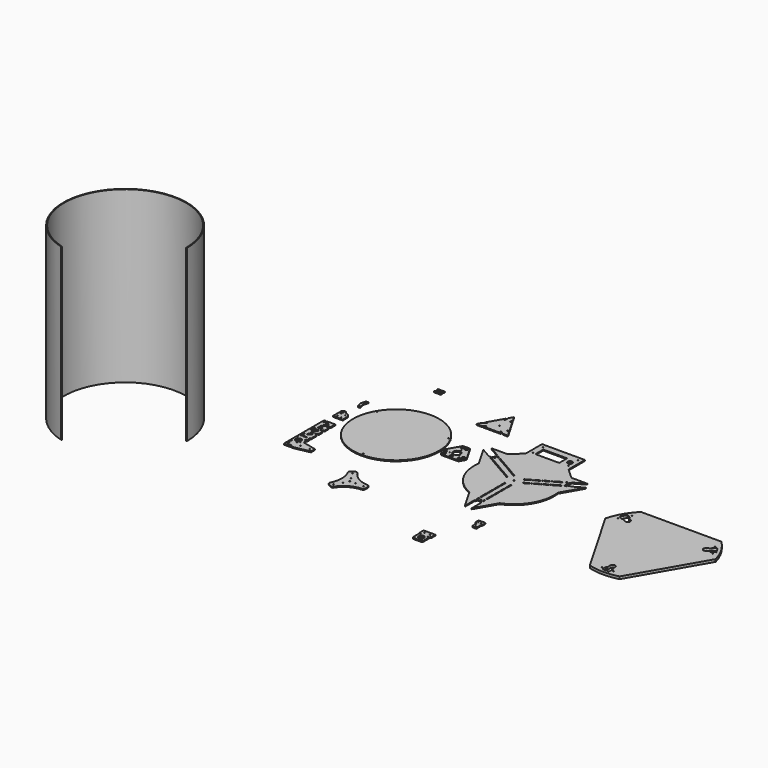
from build123d import *

# Parameters (mm, degrees)
F0_R      = 1.49999625
F0_R_2    = 1.999995
F0_R_3    = 11.4999712501
F0_W      = 3.999994
F0_H      = 4.6031024922
F0_R_4    = 4.49998875
F1_DEPTH  = 4
F0_R_5    = 177.4995562511
F0_W_2    = 3.99999
F0_H_2    = 9.9561866095
F0_R_6    = 2
F0_W_3    = 19.9999510001
F0_H_3    = 3.4640928398
F0_W_4    = 3.999988
F0_H_4    = 7.9999760001
F0_R_7    = 1.9999942213
F0_W_5    = 4
F0_H_5    = 29.9999350002
F0_H_6    = 19.9999400001
F0_H_7    = 19.9999410001
F0_H_8    = 23.1915490211
F0_R_8    = 2.4999934422
F0_R_9    = 1.9999957017
F0_R_10   = 1.75
F0_R_11   = 1.9999950064
F0_R_12   = 10
F0_R_13   = 1.9999769978
F0_R_14   = 1.9999882693
F0_R_15   = 2.0033655233
F0_R_16   = 1.4940821477
F0_R_17   = 1.9930891667
F2_R      = 2
F2_R_2    = 1.5
F3_DEPTH  = 4
F4_R      = 5.9
F4_R_2    = 1.5
F4_R_3    = 6
F4_R_4    = 15
F5_DEPTH  = 4
F7_DEPTH  = 40
F9_DEPTH  = 700
F10_R     = 2
F11_DEPTH = 10
F12_R     = 1.5
F12_R_2   = 2
F14_DEPTH = 4
F13_R     = 1.6499986081
F13_R_2   = 11.0499960842
F13_R_3   = 2


# Not quite as in the source:
# - ends of sketch curves that miss each other by under 0.0002 mm in the source are joined


with BuildPart() as f1:
    # F0 (on Top) → F1 (new body)
    with BuildSketch(Plane.XY):
        Polygon((-439.5795490511, -125.5086882283), (-439.6210259474, -125.4915762711), (-440.7988980027, -125.4915762711), (-440.7988980027, -122.491583771), (-439.1989020027, -122.491583771), (-439.1989020027, -122.5621985945), (-439.1938570154, -122.5615335962), (-439.1955270112, -120.5603685991), (-435.9955370112, -120.5576966058), (-435.9938640153, -122.5615335962), (-432.9989175027, -122.5615335962), (-432.9989175027, -118.6865432836), (-428.9989275027, -118.6865432836), (-428.9989275027, -95.4949932625), (-464.8342439144, -95.4949932625), (-464.8342439144, -106.9297106757), (-468.8342339144, -106.9297106757), (-468.8342339144, -95.4949932625), (-474.998812503, -95.4949932625), (-474.998812503, -302.9560376099), (-432.9989175027, -302.9560376099), (-372.9990675023, -290.4291429271), (-372.9990675023, -270.429192927), (-428.9989275027, -257.2412538969), (-428.9989275027, -249.2412738968), (-432.9989175027, -249.2412738968), (-432.9989175027, -238.816799958), (-428.9989275027, -238.816799958), (-428.9989275027, -230.8168199579), (-432.9989175027, -230.8168199579), (-432.9989175027, -220.9362876593), (-428.9989275027, -220.9362876593), (-428.9989275027, -190.9363626591), (-432.9989175027, -190.9363626591), (-432.9989175027, -187.0613723466), (-435.9400231499, -187.0563143592), (-435.9441941395, -189.0601753496), (-439.1441871395, -189.0601753496), (-439.1400291499, -187.0664223339), (-440.7322311694, -187.0664223339), (-440.7322311694, -184.0664298339), (-439.1808460479, -184.0664298339), (-439.1425161437, -184.0613798465), (-439.1441871395, -182.0601928495), (-435.9441941395, -182.0601928495), (-435.9425231437, -184.0613798465), (-432.9989175027, -184.0613798465), (-432.9989175027, -180.186389534), (-428.9989275027, -180.186389534), (-428.9989275027, -160.1864395339), (-432.9989175027, -160.1864395339), (-432.9989175027, -156.3114492214), (-435.9656930858, -156.306413234), (-435.9640200899, -158.3102612243), (-439.16401409, -158.3102612243), (-439.1656840858, -156.3090842273), (-439.236808908, -156.2998332504), (-440.7655640861, -156.2998332504), (-440.7655640861, -153.2998407504), (-439.1681960795, -153.2998407504), (-439.1698570754, -151.3102807243), (-435.9698640753, -151.3102807243), (-435.9681930795, -153.3114567214), (-432.9989175027, -153.3114567214), (-432.9989175027, -149.4364664088), (-428.9989275027, -149.4364664088), (-428.9989275027, -129.4365164087), (-432.9989175027, -129.4365164087), (-432.9989175027, -125.5615260962), (-435.9913630216, -125.5565111087), (-435.9896930258, -127.5576771058), (-439.1896840258, -127.5603480991), (-439.1913540216, -125.559183102), align=None)
        with BuildLine():
            add(Edge.make_bspline(
                [(-445.5863090342, -297.4957282607), (-445.5863090342, -294.0828727047), (-459.7051392371, -295.7893004827), (-473.8239694401, -297.4957282607), (-459.7051392371, -299.2021560387), (-445.5863090342, -300.9085838167), (-445.5863090342, -297.4957282607)],
                knots=[0, 0, 0, 2.0943951024, 2.0943951024, 4.1887902048, 4.1887902048, 6.2831853072, 6.2831853072, 6.2831853072], degree=2, weights=[1, 0.5, 1, 0.5, 1, 0.5, 1]))
        make_face(mode=Mode.SUBTRACT)
        with Locations((-469.552397119, -291.3865105337)):
            Circle(F0_R, mode=Mode.SUBTRACT)
        with Locations((-438.4448498879, -291.3865105337)):
            Circle(F0_R, mode=Mode.SUBTRACT)
        with Locations((-469.4988262529, -280.6365374087)):
            Circle(F0_R_2, mode=Mode.SUBTRACT)
        with Locations((-469.5517851205, -268.9985985035)):
            Circle(F0_R, mode=Mode.SUBTRACT)
        with Locations((-448.2801512996, -268.9919315202)):
            Circle(F0_R, mode=Mode.SUBTRACT)
        with Locations((-423.4178604553, -280.6365374087)):
            Circle(F0_R_2, mode=Mode.SUBTRACT)
        with Locations((-386.1206556984, -280.6365374087)):
            Circle(F0_R_2, mode=Mode.SUBTRACT)
        with Locations((-453.844811388, -253.5207241982)):
            Circle(F0_R_3, mode=Mode.SUBTRACT)
        with Locations((-439.7278266804, -262.5266596833)):
            Circle(F0_R, mode=Mode.SUBTRACT)
        with Locations((-469.5258531854, -237.9090702273)):
            Circle(F0_R, mode=Mode.SUBTRACT)
        with Locations((-438.4448498879, -237.9631240922)):
            Circle(F0_R, mode=Mode.SUBTRACT)
        with Locations((-467.4761833095, -222.8868237829)):
            Rectangle(F0_W, F0_H, mode=Mode.SUBTRACT)
        with BuildLine():
            add(Edge.make_bspline(
                [(-442.6737393156, -222.7585111037), (-442.6737393156, -219.3456555477), (-456.7925695186, -221.0520833257), (-470.9113997215, -222.7585111037), (-456.7925695186, -224.4649388817), (-442.6737393156, -226.1713666597), (-442.6737393156, -222.7585111037)],
                knots=[0, 0, 0, 2.0943951024, 2.0943951024, 4.1887902048, 4.1887902048, 6.2831853072, 6.2831853072, 6.2831853072], degree=2, weights=[1, 0.5, 1, 0.5, 1, 0.5, 1]))
        make_face(mode=Mode.SUBTRACT)
        with Locations((-467.4988312529, -214.9663525841)):
            Circle(F0_R, mode=Mode.SUBTRACT)
        Polygon((-469.4761793095, -205.1884330289), (-465.4761863095, -205.1884330289), (-465.4761863095, -209.8352954118), (-469.4761803095, -209.8352954118), align=None, mode=Mode.SUBTRACT)
        Polygon((-451.9988700028, -205.9363251592), (-461.4988462529, -205.9363251592), (-452.1737155657, -195.9363501591), (-451.9988700028, -195.9363501591), (-451.9814170465, -195.7301356747), (-447.2921947695, -190.7015612461), (-442.4988937528, -195.9363501591), align=None, mode=Mode.SUBTRACT)
        with Locations((-451.9988700028, -185.5664260839)):
            Circle(F0_R_4, mode=Mode.SUBTRACT)
        Polygon((-465.5654720863, -167.7282536794), (-465.5654720863, -172.3313561716), (-469.5654650863, -172.3313561716), (-469.5654660863, -167.7282536794), align=None, mode=Mode.SUBTRACT)
        with Locations((-467.5654690863, -162.2343414141)):
            Circle(F0_R, mode=Mode.SUBTRACT)
        Polygon((-456.7275011812, -180.397214007), (-461.4988462529, -175.186402034), (-451.9988700028, -165.1864270339), (-461.4988462529, -165.1864270339), (-456.7488581278, -159.9989750026), (-447.3363046592, -159.9989750026), (-442.6737393156, -165.1864270339), align=None, mode=Mode.SUBTRACT)
        Polygon((-469.5654650863, -152.3314141715), (-465.5654720863, -152.3314141715), (-465.5654720863, -156.9782765543), (-469.5654660863, -156.9782765543), align=None, mode=Mode.SUBTRACT)
        Polygon((-456.7055452361, -129.2017149957), (-442.4988937528, -144.4364789088), (-447.2488818778, -149.62400094), (-456.7488581278, -149.62400094), (-461.4988462529, -144.4364789088), (-451.9988700028, -144.4364789088), (-461.4988462529, -134.4365039087), align=None, mode=Mode.SUBTRACT)
        with Locations((-451.9988700028, -123.991580021)):
            Circle(F0_R_4, mode=Mode.SUBTRACT)
        Polygon((-451.8240234399, -103.6865807835), (-442.4988937528, -113.6865557836), (-447.2921947695, -118.9213456966), (-461.4988462529, -103.6865807835), align=None, mode=Mode.SUBTRACT)
    extrude(amount=F1_DEPTH)


with BuildPart() as f1b:
    # F0 (on Top) → F1, piece 2 (new body)
    with BuildSketch(Plane.XY):
        with Locations((-231.1251601871, -29.9759380602)):
            Circle(F0_R_5)
        with Locations((-231.1251601871, -199.2255149362)):
            Circle(F0_R_2, mode=Mode.SUBTRACT)
        with Locations((-378.5313116717, 55.8541043647)):
            Circle(F0_R_2, mode=Mode.SUBTRACT)
        with Locations((-83.6997907505, 56.0153949615)):
            Circle(F0_R_2, mode=Mode.SUBTRACT)
    extrude(amount=F1_DEPTH)


with BuildPart() as f1c:
    # F0 (on Top) → F1, piece 3 (new body)
    with BuildSketch(Plane.XY):
        Polygon((-442.7478361304, 91.5328801678), (-451.8370994072, 91.5328801678), (-457.283592791, 71.5697730756), (-451.8370994072, 49.5329861675), (-442.7478361304, 49.5329861493), (-448.1943295142, 71.5697720756), align=None)
        with Locations((-448.8326909183, 54.9859315352)):
            Circle(F0_R, mode=Mode.SUBTRACT)
        with Locations((-448.7918990202, 86.0799338002)):
            Circle(F0_R, mode=Mode.SUBTRACT)
    extrude(amount=F1_DEPTH)


with BuildPart() as f1d:
    # F0 (on Top) → F1, piece 4 (new body)
    with BuildSketch(Plane.XY):
        Polygon((-312.8262449344, 291.4364354089), (-314.8593918515, 291.4364354089), (-314.8610558474, 289.4432753918), (-318.0610468474, 289.4459463851), (-318.0593768516, 291.4471123822), (-321.0518233704, 291.4420963948), (-321.0518233704, 287.5671060822), (-324.999187502, 287.5671060822), (-324.999187502, 282.9560946098), (-296.999187502, 282.9560946098), (-296.999187502, 287.5671060822), (-300.9465516336, 287.5671060822), (-300.9465516336, 291.4420963948), (-303.9389981525, 291.4471123822), (-303.9373281567, 289.4459463851), (-303.9431711421, 289.4459415081), (-303.9431711421, 289.4432753918), (-307.1373191567, 289.4432753918), (-307.1373191567, 296.4432597708), (-307.1373191567, 296.4459268852), (-303.9431711421, 296.4459268852), (-303.9414991462, 294.4420888948), (-303.9389981525, 294.4420888948), (-300.9465516336, 294.4420888948), (-300.9465516336, 298.3170792073), (-296.999187502, 298.3170792073), (-296.999187502, 302.9560946098), (-324.999187502, 302.9560946098), (-324.999187502, 298.3171372072), (-321.0518233704, 298.3170792073), (-321.0518233704, 294.4420888948), (-318.0568758578, 294.4420888948), (-318.055203862, 296.4459268852), (-314.855212862, 296.4432548919), (-314.8568828578, 294.4420888948), (-314.8139219652, 294.4364279089), (-312.8262449344, 294.4364279089), align=None)
        Polygon((-307.1414921463, 294.4420888948), (-307.1414921463, 291.4364354089), (-309.1721300697, 291.4364354089), (-309.1721300697, 294.4364279089), (-309.1721300697, 294.4420888948), align=None, mode=Mode.SUBTRACT)
    extrude(amount=F1_DEPTH)


with BuildPart() as f1e:
    # F0 (on Top) → F1, piece 5 (new body)
    with BuildSketch(Plane.XY):
        Polygon((-1.8421003947, 285.6355719111), (-11.8420763948, 302.9560366099), (-21.8420513949, 285.6355719111), (-21.8420513949, 272.2152924618), (-1.8421003947, 272.2152924618), align=None)
        Polygon((16.4874262814, 195.434410914), (18.4874214067, 198.8985040612), (9.8651113372, 203.8765973085), (7.8651163372, 200.4125039687), align=None)
        Polygon((28.4873965199, 216.2189689089), (30.4873917815, 219.6830622923), (21.8650813373, 224.6611553471), (19.8650863373, 221.1970620073), align=None)
        with Locations((0.1578946053, 263.7731063172)):
            Rectangle(F0_W_2, F0_H_2)
        Polygon((-1.8421003947, 258.7950130125), (-1.8421003947, 268.751199622), (-21.8420513949, 268.751199622), (-21.8420513949, 258.7950130125), (-25.8420413949, 258.7950130125), (-25.8420413949, 268.751199622), (-25.8420413949, 272.2152924618), (-25.8420413949, 278.7073862315), (-62.7938540154, 214.7049692376), (-57.1715370057, 217.9510153453), (-54.1715435711, 219.6830622923), (-45.5492331269, 224.6611553471), (-43.5492381269, 221.1970630073), (-52.1715487116, 216.2189696768), (-42.1715730107, 198.8985041684), (-33.5492631268, 203.8765973085), (-31.5492681268, 200.4125049687), (-40.1715780711, 195.434411414), (-43.1715704387, 193.7023648085), (-48.7938880153, 190.4563178592), (25.1097362257, 190.4563178592), (19.4874189347, 193.7023643176), (16.4874262814, 195.434410914), (7.8651163372, 200.4125039687), (9.8651113372, 203.8765973085), (18.4874214067, 198.8985040612), (28.4873965199, 216.2189689089), (19.8650863373, 221.1970620073), (21.8650813373, 224.6611553471), (30.4873917815, 219.6830622923), (33.4873845882, 217.9510157079), (39.1097022257, 214.7049692376), (2.1578896053, 278.7073862315), (2.1578896053, 272.2152924618), (2.1578896053, 268.751199622), (2.1578896053, 258.7950130125), align=None)
        with Locations((-11.8420758948, 227.9562243465)):
            Circle(F0_R_6, mode=Mode.SUBTRACT)
        with Locations((-23.8420463949, 263.7731063172)):
            Rectangle(F0_W_2, F0_H_2)
        Polygon((-45.1715655711, 197.1664575839), (-55.1715419814, 214.4869227571), (-66.7938440154, 207.776783558), (-76.7938190155, 190.4563178592), (-56.7938680153, 190.4563178592), align=None)
        Polygon((-45.5492331269, 224.6611553471), (-54.1715435711, 219.6830622923), (-52.1715487116, 216.2189696768), (-43.5492381269, 221.1970630073), align=None)
        Polygon((-33.5492631268, 203.8765973085), (-42.1715730107, 198.8985041684), (-40.1715780711, 195.434411414), (-31.5492681268, 200.4125049687), align=None)
        Polygon((43.1096922258, 207.776782558), (31.4873892815, 214.4869222827), (21.4874140575, 197.1664574245), (33.1097162257, 190.4563178592), (53.1096672258, 190.4563178592), align=None)
        Polygon((21.4874140575, 197.1664574245), (31.4873892815, 214.4869222827), (28.4873965199, 216.2189689089), (18.4874214067, 198.8985040612), align=None)
        with Locations((-11.8420758948, 270.4832460419)):
            Rectangle(F0_W_3, F0_H_3)
        Polygon((-52.1715487116, 216.2189696768), (-55.1715419814, 214.4869227571), (-45.1715655711, 197.1664575839), (-42.1715730107, 198.8985041684), align=None)
    extrude(amount=F1_DEPTH)


with BuildPart() as f1f:
    # F0 (on Top) → F1, piece 6 (new body)
    with BuildSketch(Plane.XY):
        with BuildLine():
            Line((131.7235082388, 88.5993365017), (66.7513821215, 88.5993365017))
            Line((66.7513821215, 88.5993365017), (111.0197374507, 63.0409903975))
            Line((111.0197374507, 63.0409903975), (109.0197424506, 59.5768970578))
            Line((109.0197424506, 59.5768970578), (115.1252134995, 56.0519168039))
            Line((115.1252134995, 56.0519168039), (105.1252384995, 38.7314511051))
            Line((105.1252384995, 38.7314511051), (99.0197737631, 42.2564432926))
            Line((99.0197737631, 42.2564432926), (97.0197787631, 38.7923499528))
            Line((97.0197787631, 38.7923499528), (52.7514171215, 64.3506861233))
            Line((52.7514171215, 64.3506861233), (100.9852385369, -19.1927430181))
            ThreePointArc((100.9852385369, -19.1927430181), (121.3444904617, -123.6659645283), (201.6413278967, -193.5342051645))
            Line((201.6413278967, -193.5342051645), (249.8751493121, -277.0776343059))
            Line((249.8751493121, -277.0776343059), (249.8751493121, -225.9609400976))
            Line((249.8751493121, -225.9609400976), (253.8751393121, -225.9609400976))
            Line((253.8751393121, -225.9609400976), (253.8751393121, -218.9109567226))
            Line((253.8751393121, -218.9109567226), (273.8750893123, -218.9109567226))
            Line((273.8750893123, -218.9109567226), (273.8750893123, -225.9609400976))
            Line((273.8750893123, -225.9609400976), (277.8750793123, -225.9609400976))
            Line((277.8750793123, -225.9609400976), (277.8750793123, -277.0776343059))
            Line((277.8750793123, -277.0776343059), (326.1089007277, -193.5342051645))
            ThreePointArc((326.1089007277, -193.5342051645), (406.4100868046, -123.6684751011), (426.7649910875, -19.1927430181))
            Line((426.7649910875, -19.1927430181), (474.998812503, 64.3506861233))
            Line((474.998812503, 64.3506861233), (430.7304571739, 38.7923390192))
            Line((430.7304571739, 38.7923390192), (428.7304621738, 42.2564323589))
            Line((428.7304621738, 42.2564323589), (422.6249974375, 38.7314401714))
            Line((422.6249974375, 38.7314401714), (412.6250224374, 56.0519058702))
            Line((412.6250224374, 56.0519058702), (418.7304871738, 59.5768970578))
            Line((418.7304871738, 59.5768970578), (416.7304921738, 63.0409903975))
            Line((416.7304921738, 63.0409903975), (460.9988465029, 88.5993365017))
            Line((460.9988465029, 88.5993365017), (396.0267213856, 88.5993365017))
            Line((396.0267213856, 88.5993365017), (352.1159646784, 128.1467825174))
            Line((352.1159646784, 128.1467825174), (352.1159646784, 212.6197069883))
            Line((352.1159646784, 212.6197069883), (175.634264946, 212.6197069883))
            Line((175.634264946, 212.6197069883), (175.634264946, 128.1467825174))
            Line((175.634264946, 128.1467825174), (131.7235082388, 88.5993365017))
        make_face()
        with Locations((251.8751113122, -211.5364981588)):
            Rectangle(F0_W_4, F0_H_4, mode=Mode.SUBTRACT)
        with Locations((263.8751143122, -211.5364761588)):
            Circle(F0_R_7, mode=Mode.SUBTRACT)
        with Locations((275.8750793123, -211.5364771588)):
            Rectangle(F0_W_4, F0_H_4, mode=Mode.SUBTRACT)
        with Locations((251.8751443121, -182.65599636)):
            Rectangle(F0_W_5, F0_H_5, mode=Mode.SUBTRACT)
        with Locations((275.8750793123, -182.65599636)):
            Rectangle(F0_W_4, F0_H_5, mode=Mode.SUBTRACT)
        with Locations((251.8751443121, -162.2810432974)):
            Circle(F0_R_6, mode=Mode.SUBTRACT)
        with Locations((275.8750793123, -162.2810432974)):
            Circle(F0_R_6, mode=Mode.SUBTRACT)
        with Locations((206.4286084064, -22.0654858745)):
            Circle(F0_R_6, mode=Mode.SUBTRACT)
        Polygon((210.0834857913, -26.4850257874), (212.0834807913, -23.0209324477), (232.1679543738, -34.6167053514), (230.1679575801, -38.080800798), align=None, mode=Mode.SUBTRACT)
        Polygon((183.4532703668, -11.1100642248), (185.4532653668, -7.6459708851), (202.7737310657, -17.6459458851), (200.7737360657, -21.1100392249), align=None, mode=Mode.SUBTRACT)
        with Locations((179.798393129, -6.6905240572)):
            Circle(F0_R_6, mode=Mode.SUBTRACT)
        Polygon((222.0834571602, -5.7004653779), (224.0834521603, -2.2363720381), (244.1679225802, -13.8321504196), (242.1679275802, -17.2962427594), align=None, mode=Mode.SUBTRACT)
        with Locations((218.4285798248, -1.2809253793)):
            Circle(F0_R_6, mode=Mode.SUBTRACT)
        with Locations((251.8751443121, -146.9060877348)):
            Rectangle(F0_W_5, F0_H_6, mode=Mode.SUBTRACT)
        with Locations((275.8750793123, -146.9060877348)):
            Rectangle(F0_W_4, F0_H_6, mode=Mode.SUBTRACT)
        with Locations((251.8751443121, -131.5311201722)):
            Circle(F0_R_6, mode=Mode.SUBTRACT)
        with Locations((251.8751443121, -116.1561521096)):
            Rectangle(F0_W_5, F0_H_7, mode=Mode.SUBTRACT)
        with Locations((275.8750793123, -131.5311201722)):
            Circle(F0_R_6, mode=Mode.SUBTRACT)
        with Locations((275.8750793123, -116.1561521096)):
            Rectangle(F0_W_4, F0_H_7, mode=Mode.SUBTRACT)
        with Locations((251.8751443121, -100.781196047)):
            Circle(F0_R_6, mode=Mode.SUBTRACT)
        with Locations((275.8750793123, -100.781196047)):
            Circle(F0_R_6, mode=Mode.SUBTRACT)
        with Locations((251.8751443121, -83.8104359739)):
            Rectangle(F0_W_5, F0_H_8, mode=Mode.SUBTRACT)
        with Locations((275.8750793123, -83.8104359739)):
            Rectangle(F0_W_4, F0_H_8, mode=Mode.SUBTRACT)
        with Locations((263.8751148122, -41.3758700603)):
            Circle(F0_R_8, mode=Mode.SUBTRACT)
        Polygon((283.5823070442, -13.8321504196), (303.666778833, -2.2363754091), (305.6667738331, -5.7004677488), (285.5823020442, -17.2962427594), align=None, mode=Mode.SUBTRACT)
        Polygon((295.5822770443, -34.6167084582), (315.6667488331, -23.0209324477), (317.6667438331, -26.4850257874), (297.5822720443, -38.080800798), align=None, mode=Mode.SUBTRACT)
        with Locations((321.3216211994, -22.0654858423)):
            Circle(F0_R_6, mode=Mode.SUBTRACT)
        with Locations((309.3216511993, -1.2809283037)):
            Circle(F0_R_6, mode=Mode.SUBTRACT)
        Polygon((326.9764935588, -21.1100392249), (324.9764985587, -17.6459458851), (342.2969632576, -7.6459708851), (344.2969582576, -11.1100642248), align=None, mode=Mode.SUBTRACT)
        with Locations((347.9518356204, -6.6905242737)):
            Circle(F0_R_6, mode=Mode.SUBTRACT)
        Polygon((114.9758125605, 33.0442053895), (112.9758175605, 29.5801120497), (106.0476318809, 33.5801020497), (108.0476268809, 37.0441953895), align=None, mode=Mode.SUBTRACT)
        with Locations((116.5117067207, 43.7044327389)):
            Circle(F0_R_9, mode=Mode.SUBTRACT)
        Polygon((123.5326041685, 28.1039387402), (149.5133012167, 13.1039772401), (147.5133062167, 9.6398839003), (121.5326091685, 24.6398464004), align=None, mode=Mode.SUBTRACT)
        with Locations((153.1681786016, 8.6844373271)):
            Circle(F0_R_6, mode=Mode.SUBTRACT)
        Polygon((176.1435156412, -2.2709843225), (174.1435206412, -5.7350776623), (156.8230559424, 4.2648973378), (158.8230509424, 7.7289906775), align=None, mode=Mode.SUBTRACT)
        with Locations((165.1681505852, 29.4689988013)):
            Circle(F0_R_6, mode=Mode.SUBTRACT)
        Polygon((197.4532363669, 13.1385871535), (214.7737010657, 3.1386121535), (212.7737075016, -0.3254786258), (195.4532413669, 9.6744938138), align=None, mode=Mode.SUBTRACT)
        with Locations((191.79836558, 14.0940364945)):
            Circle(F0_R_6, mode=Mode.SUBTRACT)
        Polygon((170.8230209424, 28.5135487161), (188.1434866413, 18.5135737161), (186.1434933597, 15.0494834263), (168.8230259424, 25.0494553764), align=None, mode=Mode.SUBTRACT)
        Polygon((135.5325741686, 48.8884967788), (161.5132712168, 33.8885352787), (159.5132782179, 30.4244454784), (133.5325791686, 45.424404439), align=None, mode=Mode.SUBTRACT)
        Polygon((118.047601881, 54.3646600883), (120.047596881, 57.8287534281), (126.9757873939, 53.8287717997), (124.9757875605, 50.3646700883), align=None, mode=Mode.SUBTRACT)
        with Locations((191.1711761168, 146.9972811108)):
            Circle(F0_R_10, mode=Mode.SUBTRACT)
        Polygon((314.9765235587, -0.3254811863), (312.9765285587, 3.1386111535), (330.2969932575, 13.1385861535), (332.2969882575, 9.6744938138), align=None, mode=Mode.SUBTRACT)
        with Locations((335.9518656203, 14.0940332649)):
            Circle(F0_R_6, mode=Mode.SUBTRACT)
        Polygon((341.6067379832, 15.0494803763), (339.6067429831, 18.5135727161), (356.927207682, 28.5135477161), (358.927202682, 25.0494553764), align=None, mode=Mode.SUBTRACT)
        Polygon((353.6067079832, -5.7350776623), (351.6067129832, -2.2709843225), (368.9271776821, 7.7289906775), (370.9271726821, 4.2648973378), align=None, mode=Mode.SUBTRACT)
        with Locations((374.5820500414, 8.6844372949)):
            Circle(F0_R_6, mode=Mode.SUBTRACT)
        Polygon((378.2369274077, 13.1039772401), (404.2176244559, 28.1039387402), (406.2176194559, 24.6398464004), (380.2369224077, 9.6398839003), align=None, mode=Mode.SUBTRACT)
        with Locations((362.5820800413, 29.4689948335)):
            Circle(F0_R_6, mode=Mode.SUBTRACT)
        Polygon((419.7026027435, 37.0441953895), (421.7025977435, 33.5801020497), (414.774412064, 29.5801120497), (412.774417064, 33.0442053895), align=None, mode=Mode.SUBTRACT)
        Polygon((368.2369524076, 30.4244419389), (366.2369574076, 33.8885342787), (392.2176518071, 48.8885013665), (394.2176494559, 45.424404439), align=None, mode=Mode.SUBTRACT)
        with Locations((411.2385224037, 43.7044327389)):
            Circle(F0_R_11, mode=Mode.SUBTRACT)
        Polygon((402.7744420639, 50.3646700883), (400.7744470639, 53.8287634281), (407.7026327434, 57.8287534281), (409.7026277434, 54.3646600883), align=None, mode=Mode.SUBTRACT)
        with Locations((336.3553861168, 146.9972811108)):
            Circle(F0_R_10, mode=Mode.SUBTRACT)
        with Locations((191.3553861168, 196.9446491108)):
            Circle(F0_R_10, mode=Mode.SUBTRACT)
        Polygon((300.6485231095, 185.6192490275), (300.350809158, 144.8960076725), (202.150809158, 144.8960076725), (202.4485231095, 185.6192490275), align=None, mode=Mode.SUBTRACT)
        with Locations((326.0473194219, 168.8628891764)):
            Circle(F0_R_12, mode=Mode.SUBTRACT)
        with Locations((336.3553861168, 196.9972811108)):
            Circle(F0_R_10, mode=Mode.SUBTRACT)
    extrude(amount=F1_DEPTH)


with BuildPart() as f1g:
    # F0 (on Top) → F1, piece 7 (new body)
    with BuildSketch(Plane.XY):
        with BuildLine():
            Line((-431.8410253974, -53.4667563331), (-431.8410253974, -33.466806333))
            ThreePointArc((-431.8410253974, -33.466806333), (-437.6988751291, -19.3247060645), (-451.8409753976, -13.4668563329))
            ThreePointArc((-451.8409753976, -13.4668563329), (-461.7902973253, -4.6085405914), (-471.8277604306, -13.3668565829))
            Line((-471.8277604306, -13.3668565829), (-471.8409253977, -13.4668563329))
            Line((-471.8409253977, -13.4668563329), (-471.8409253977, -53.4667563331))
            Line((-471.8409253977, -53.4667563331), (-431.8410253974, -53.4667563331))
        make_face()
        with Locations((-461.840950873, -43.4667625831)):
            Circle(F0_R_13, mode=Mode.SUBTRACT)
        with Locations((-445.8659251778, -43.4667725675)):
            Circle(F0_R_14, mode=Mode.SUBTRACT)
        with Locations((-461.840950873, -23.4747163132)):
            Circle(F0_R_15, mode=Mode.SUBTRACT)
        with Locations((-443.8431728921, -25.5569271077)):
            Circle(F0_R_16, mode=Mode.SUBTRACT)
        with Locations((-461.840950873, -13.4589708526)):
            Circle(F0_R_17, mode=Mode.SUBTRACT)
    extrude(amount=F1_DEPTH)


with BuildPart() as f3:
    # F2 (on Top) → F3 (new body)
    with BuildSketch(Plane.XY):
        with BuildLine():
            Line((-173.3191576007, -312.3464409502), (-185.7394526007, -319.5173019502))
            ThreePointArc((-185.7394526007, -319.5173019502), (-189.5272888895, -324.3374721499), (-188.9380147581, -330.4394800316))
            ThreePointArc((-188.9380147581, -330.4394800316), (-177.8813236007, -375.8740039502), (-188.9380148359, -421.3085278286))
            ThreePointArc((-188.9380148359, -421.3085278286), (-189.5272888895, -427.4105357506), (-185.7394525664, -432.2307058908))
            Line((-185.7394525664, -432.2307058908), (-173.3191576007, -439.4015669502))
            ThreePointArc((-173.3191576007, -439.4015669502), (-167.2508489819, -440.2718443354), (-162.2609918166, -436.7105138119))
            ThreePointArc((-162.2609918166, -436.7105138119), (-128.4418856195, -404.4178770248), (-83.566088559, -391.2759908533))
            ThreePointArc((-83.566088559, -391.2759908533), (-77.9869574035, -388.7353126425), (-75.7064856007, -383.0448649502))
            Line((-75.7064856007, -383.0448649502), (-75.7064856007, -368.7031429502))
            ThreePointArc((-75.7064856007, -368.7031429502), (-77.9869574035, -363.012695258), (-83.5660885958, -360.4720178441))
            ThreePointArc((-83.5660885958, -360.4720178441), (-128.4418856195, -347.3301308757), (-162.2609917909, -315.0374940721))
            ThreePointArc((-162.2609917909, -315.0374940721), (-167.2508489819, -311.476163565), (-173.3191576007, -312.3464409502))
        make_face()
        with Locations((-172.9373796007, -424.3985879502)):
            Circle(F2_R, mode=Mode.SUBTRACT)
        with Locations((-156.9805416007, -419.5396239502)):
            Circle(F2_R_2, mode=Mode.SUBTRACT)
        with Locations((-176.9547986007, -408.0074809502)):
            Circle(F2_R_2, mode=Mode.SUBTRACT)
        with Locations((-161.4547986007, -381.1606929502)):
            Circle(F2_R_2, mode=Mode.SUBTRACT)
        with Locations((-156.4575676007, -395.8547149502)):
            Circle(F2_R, mode=Mode.SUBTRACT)
        with Locations((-141.4805416007, -392.6928359502)):
            Circle(F2_R_2, mode=Mode.SUBTRACT)
        with Locations((-144.9216986007, -375.8740039502)):
            Circle(F2_R, mode=Mode.SUBTRACT)
        with Locations((-132.0091126007, -387.3950559502)):
            Circle(F2_R_2, mode=Mode.SUBTRACT)
        with Locations((-121.8499606007, -375.8740039502)):
            Circle(F2_R, mode=Mode.SUBTRACT)
        with Locations((-101.0091126007, -387.3950559502)):
            Circle(F2_R_2, mode=Mode.SUBTRACT)
        with Locations((-88.8903356007, -375.8740039502)):
            Circle(F2_R, mode=Mode.SUBTRACT)
        with Locations((-161.3317336007, -370.5705259502)):
            Circle(F2_R_2, mode=Mode.SUBTRACT)
        with Locations((-176.8317336007, -343.7237389502)):
            Circle(F2_R_2, mode=Mode.SUBTRACT)
        with Locations((-156.4575676007, -355.8932929502)):
            Circle(F2_R, mode=Mode.SUBTRACT)
        with Locations((-141.3574766007, -359.0383839502)):
            Circle(F2_R_2, mode=Mode.SUBTRACT)
        with Locations((-172.9373796007, -327.3494199502)):
            Circle(F2_R, mode=Mode.SUBTRACT)
        with Locations((-156.8574766007, -332.1915959502)):
            Circle(F2_R_2, mode=Mode.SUBTRACT)
        with Locations((-132.0091126007, -364.3307699502)):
            Circle(F2_R_2, mode=Mode.SUBTRACT)
        with Locations((-101.0091126007, -364.3307699502)):
            Circle(F2_R_2, mode=Mode.SUBTRACT)
        with Locations((-176.9547986007, -408.0074809502)):
            Circle(F2_R_2)
        with Locations((-161.4547986007, -381.1606929502)):
            Circle(F2_R_2)
        with Locations((-161.3317336007, -370.5705259502)):
            Circle(F2_R_2)
        with Locations((-132.0091126007, -364.3307699502)):
            Circle(F2_R_2)
        with Locations((-132.0091126007, -387.3950559502)):
            Circle(F2_R_2)
        with Locations((-141.4805416007, -392.6928359502)):
            Circle(F2_R_2)
        with Locations((-101.0091126007, -364.3307699502)):
            Circle(F2_R_2)
        with Locations((-101.0091126007, -387.3950559502)):
            Circle(F2_R_2)
        with Locations((-141.3574766007, -359.0383839502)):
            Circle(F2_R_2)
        with Locations((-156.9805416007, -419.5396239502)):
            Circle(F2_R_2)
        with Locations((-176.8317336007, -343.7237389502)):
            Circle(F2_R_2)
        with Locations((-156.8574766007, -332.1915959502)):
            Circle(F2_R_2)
    extrude(amount=F3_DEPTH)


with BuildPart() as f5:
    # F4 (on Top) → F5 (new body)
    with BuildSketch(Plane.XY):
        with BuildLine():
            ThreePointArc((-48.2087481727, -14.7499999003), (-49.280545, -18.75), (-48.2087481727, -22.7500000997))
            Line((-48.2087481727, -22.7500000997), (-38.393793, -39.75))
            ThreePointArc((-38.393793, -39.75), (-35.4655899501, -42.6782032591), (-31.46559, -43.75))
            Line((-31.46559, -43.75), (31.465589, -43.75))
            ThreePointArc((31.465589, -43.75), (35.4655891667, -42.6782031341), (38.3937924227, -39.7499996667))
            Line((38.3937924227, -39.7499996667), (48.208747, -22.75))
            ThreePointArc((48.208747, -22.75), (49.280544, -18.75), (48.2087471727, -14.7499999003))
            Line((48.2087471727, -14.7499999003), (16.743157, 39.75))
            ThreePointArc((16.743157, 39.75), (13.8149539501, 42.6782032591), (9.814954, 43.75))
            Line((9.814954, 43.75), (-9.814955, 43.75))
            ThreePointArc((-9.814955, 43.75), (-13.8149549501, 42.6782032591), (-16.7431581727, 39.7500000997))
            Line((-16.7431581727, 39.7500000997), (-48.2087481727, -14.7499999003))
        make_face()
        with Locations((-30, -32.707513)):
            Circle(F4_R, mode=Mode.SUBTRACT)
        with Locations((-37.912879, -19.002006)):
            Circle(F4_R, mode=Mode.SUBTRACT)
        with Locations((-19.485572, -17.5)):
            Circle(F4_R_2, mode=Mode.SUBTRACT)
        with Locations((0, -34.25)):
            Circle(F4_R_3, mode=Mode.SUBTRACT)
        with Locations((30, -32.707513)):
            Circle(F4_R, mode=Mode.SUBTRACT)
        with Locations((19.485571, -17.5)):
            Circle(F4_R_2, mode=Mode.SUBTRACT)
        with Locations((0, -6.25)):
            Circle(F4_R_4, mode=Mode.SUBTRACT)
        with Locations((37.912878, -19.002006)):
            Circle(F4_R, mode=Mode.SUBTRACT)
        with Locations((-7.912879, 32.959519)):
            Circle(F4_R, mode=Mode.SUBTRACT)
        with Locations((0, 16.25)):
            Circle(F4_R_2, mode=Mode.SUBTRACT)
        with Locations((7.912878, 32.959519)):
            Circle(F4_R, mode=Mode.SUBTRACT)
    extrude(amount=F5_DEPTH)


with BuildPart() as f7:
    # F6 (on Top) → F7 (new body)
    with BuildSketch(Plane.XY):
        with BuildLine():
            ThreePointArc((-1047.5159788132, -146.9914472103), (-1022.1316342056, -149.4472177623), (-997.1604939163, -154.6277498596))
            Line((-997.1604939163, -154.6277498596), (-993.6036226722, -145.2269445211))
            ThreePointArc((-993.6036226722, -145.2269445211), (-1057.5967746323, -136.7795008877), (-1121.5843638588, -145.2689782991))
            Line((-1121.5843638588, -145.2689782991), (-1119.5153640317, -155.0689779092))
            ThreePointArc((-1119.5153640317, -155.0689779092), (-1093.7415152966, -149.5763347538), (-1067.5159788132, -146.9914472103))
            Line((-1067.5159788132, -146.9914472103), (-1067.5159788132, -161.9914472103))
            Line((-1067.5159788132, -161.9914472103), (-1057.5159788132, -161.9914472103))
            Line((-1057.5159788132, -161.9914472103), (-1047.5159788132, -161.9914472103))
            Line((-1047.5159788132, -161.9914472103), (-1047.5159788132, -146.9914472103))
        make_face()
    extrude(amount=F7_DEPTH)


with BuildPart() as f9:
    # F8 (on Top) → F9 (new body)
    with BuildSketch(Plane.XY):
        with BuildLine():
            ThreePointArc((-1053.2840452376, -721.2824326007), (-1139.6458620334, -279.6567894281), (-736.2761964798, -479.1172742844))
            Line((-736.2761964798, -479.1172742844), (-733.2761964798, -479.1172742844))
            ThreePointArc((-733.2761964798, -479.1172742844), (-1141.4670134145, -277.2727995693), (-1054.0729836689, -724.1768368834))
            Line((-1054.0729836689, -724.1768368834), (-1053.2840452376, -721.2824326007))
        make_face()
    extrude(amount=F9_DEPTH)


with BuildPart() as f11:
    # F10 (on Top) → F11 (new body)
    with BuildSketch(Plane.XY):
        with BuildLine():
            Line((1057.4444574637, 33.5686378129), (725.9635072428, 33.5686378129))
            ThreePointArc((725.9635072428, 33.5686378129), (688.1880124633, -15.5299663543), (664.5551213544, -72.7938065576))
            Line((664.5551213544, -72.7938065576), (830.2955964634, -359.8647303169))
            ThreePointArc((830.2955964634, -359.8647303169), (891.7039823532, -368.0299663534), (953.1123682431, -359.8647303169))
            Line((953.1123682431, -359.8647303169), (1118.852843352, -72.7938065576))
            ThreePointArc((1118.852843352, -72.7938065576), (1095.2199522431, -15.5299663543), (1057.4444574637, 33.5686378129))
        make_face()
        with Locations((867.7039823532, -344.5839856931)):
            Circle(F10_R, mode=Mode.SUBTRACT)
        with BuildLine():
            Line((901.7039823532, -354.5839856931), (881.7039823532, -354.5839856931))
            Line((881.7039823532, -354.5839856931), (877.7039823532, -354.5839856931))
            Line((877.7039823532, -354.5839856931), (877.7039823532, -334.5839856931))
            Line((877.7039823532, -334.5839856931), (881.7039823532, -334.5839856931))
            Line((881.7039823532, -334.5839856931), (881.7039823532, -318.5839856931))
            ThreePointArc((881.7039823532, -318.5839856931), (891.7039823532, -308.5839856931), (901.7039823532, -318.5839856931))
            Line((901.7039823532, -318.5839856931), (901.7039823532, -334.5839856931))
            Line((901.7039823532, -334.5839856931), (905.7039823532, -334.5839856931))
            Line((905.7039823532, -334.5839856931), (905.7039823532, -354.5839856931))
            Line((905.7039823532, -354.5839856931), (901.7039823532, -354.5839856931))
        make_face(mode=Mode.SUBTRACT)
        with Locations((915.7039823532, -344.5839856951)):
            Circle(F10_R, mode=Mode.SUBTRACT)
        with Locations((696.4928273306, -48.0375663734)):
            Circle(F10_R, mode=Mode.SUBTRACT)
        with BuildLine():
            Line((694.8325732945, -30.9132107214), (704.8325732945, -13.5927026457))
            Line((704.8325732945, -13.5927026457), (706.8325732945, -10.1286010305))
            Line((706.8325732945, -10.1286010305), (724.1530813701, -20.1286010305))
            Line((724.1530813701, -20.1286010305), (722.1530813701, -23.5927026457))
            Line((722.1530813701, -23.5927026457), (736.0094878307, -31.5927026457))
            ThreePointArc((736.0094878307, -31.5927026457), (739.6697418685, -45.2529566835), (726.0094878307, -48.9132107214))
            Line((726.0094878307, -48.9132107214), (712.1530813701, -40.9132107214))
            Line((712.1530813701, -40.9132107214), (710.1530813701, -44.3773123365))
            Line((710.1530813701, -44.3773123365), (692.8325732945, -34.3773123365))
            Line((692.8325732945, -34.3773123365), (694.8325732945, -30.9132107214))
        make_face(mode=Mode.SUBTRACT)
        with Locations((720.4928273323, -6.4683469927)):
            Circle(F10_R, mode=Mode.SUBTRACT)
        with Locations((1086.9151373741, -48.0375663743)):
            Circle(F10_R, mode=Mode.SUBTRACT)
        with BuildLine():
            Line((1078.575391412, -13.5927026457), (1088.575391412, -30.9132107214))
            Line((1088.575391412, -30.9132107214), (1090.575391412, -34.3773123365))
            Line((1090.575391412, -34.3773123365), (1073.2548833363, -44.3773123365))
            Line((1073.2548833363, -44.3773123365), (1071.2548833363, -40.9132107214))
            Line((1071.2548833363, -40.9132107214), (1057.3984768757, -48.9132107214))
            ThreePointArc((1057.3984768757, -48.9132107214), (1043.7382228379, -45.2529566835), (1047.3984768757, -31.5927026457))
            Line((1047.3984768757, -31.5927026457), (1061.2548833363, -23.5927026457))
            Line((1061.2548833363, -23.5927026457), (1059.2548833363, -20.1286010305))
            Line((1059.2548833363, -20.1286010305), (1076.575391412, -10.1286010305))
            Line((1076.575391412, -10.1286010305), (1078.575391412, -13.5927026457))
        make_face(mode=Mode.SUBTRACT)
        with Locations((1062.9151373758, -6.4683469917)):
            Circle(F10_R, mode=Mode.SUBTRACT)
    extrude(amount=F11_DEPTH)


with BuildPart() as f14:
    # F12 (on Top) → F14 (new body)
    with BuildSketch(Plane.XY):
        with BuildLine():
            Line((361.1430478096, -374.1301381588), (366.1430478096, -374.1301381588))
            Line((366.1430478096, -374.1301381588), (374.1430478096, -374.1301381588))
            Line((374.1430478096, -374.1301381588), (374.1430478096, -349.1301381588))
            Line((374.1430478096, -349.1301381588), (376.6430478096, -349.1301381588))
            Line((376.6430478096, -349.1301381588), (376.6430478096, -329.1301381588))
            Line((376.6430478096, -329.1301381588), (374.1430478096, -329.1301381588))
            Line((374.1430478096, -329.1301381588), (352.5698530674, -329.1301381588))
            ThreePointArc((352.5698530674, -329.1301381588), (349.0343191615, -330.5946042529), (347.5698530674, -334.1301381588))
            Line((347.5698530674, -334.1301381588), (347.5698530674, -344.1301381588))
            ThreePointArc((347.5698530674, -344.1301381588), (349.0343191615, -347.6656720647), (352.5698530674, -349.1301381588))
            Line((352.5698530674, -349.1301381588), (355.4620707035, -349.1301381588))
            ThreePointArc((355.4620707035, -349.1301381588), (355.9435942331, -349.3295917353), (356.1430478096, -349.8111152649))
            Line((356.1430478096, -349.8111152649), (356.1430478096, -369.1301381588))
            ThreePointArc((356.1430478096, -369.1301381588), (357.6075139037, -372.6656720647), (361.1430478096, -374.1301381588))
        make_face()
        with Locations((359.6703410149, -358.1301381588)):
            Circle(F12_R, mode=Mode.SUBTRACT)
        with Locations((366.1430478096, -366.1301381588)):
            Circle(F12_R, mode=Mode.SUBTRACT)
        with Locations((366.1430478096, -356.1301381588)):
            Circle(F12_R, mode=Mode.SUBTRACT)
        with Locations((354.0793657303, -339.1301381588)):
            Circle(F12_R_2, mode=Mode.SUBTRACT)
        with Locations((366.1430478096, -339.1301381588)):
            Circle(F12_R_2, mode=Mode.SUBTRACT)
    extrude(amount=F14_DEPTH)


with BuildPart() as f14b:
    # F13 (on Top) → F14, piece 2 (new body)
    with BuildSketch(Plane.XY):
        with BuildLine():
            Line((292.7851694811, -493.9909535475), (260.7827364579, -493.9909535475))
            Line((260.7827364579, -493.9909535475), (255.7827364579, -493.9909535475))
            Line((255.7827364579, -493.9909535475), (253.2827364579, -493.9909535475))
            Line((253.2827364579, -493.9909535475), (253.2827366085, -513.9909535475))
            Line((253.2827366085, -513.9909535475), (255.7827366085, -513.9909535475))
            Line((255.7827366085, -513.9909535475), (255.7827364579, -550.9733987741))
            ThreePointArc((255.7827364579, -550.9733987741), (257.2472025519, -554.5089326801), (260.7827364579, -555.9733987741))
            Line((260.7827364579, -555.9733987741), (292.7851696929, -555.9733987741))
            ThreePointArc((292.7851696929, -555.9733987741), (296.320703606, -554.5089326728), (297.7851696929, -550.9733987537))
            Line((297.7851696929, -550.9733987537), (297.7851695422, -513.9909535475))
            Line((297.7851695422, -513.9909535475), (301.7851695422, -513.9909535475))
            Line((301.7851695422, -513.9909535475), (301.7851695422, -493.9909535475))
            Line((301.7851695422, -493.9909535475), (297.7851696929, -493.9909535475))
            Line((297.7851696929, -493.9909535475), (292.7851694811, -493.9909535475))
        make_face()
        with Locations((261.2327118, -550.5409616528)):
            Circle(F13_R, mode=Mode.SUBTRACT)
        with Locations((292.3326985525, -550.4883321528)):
            Circle(F13_R, mode=Mode.SUBTRACT)
        with Locations((276.7827099262, -534.9909626528)):
            Circle(F13_R_2, mode=Mode.SUBTRACT)
        with Locations((261.2327143045, -519.2679537436)):
            Circle(F13_R, mode=Mode.SUBTRACT)
        with Locations((292.3327068, -519.2675001528)):
            Circle(F13_R, mode=Mode.SUBTRACT)
        with Locations((265.7827364579, -503.9909535475)):
            Circle(F13_R_3, mode=Mode.SUBTRACT)
        with Locations((287.7851696929, -503.9909535475)):
            Circle(F13_R_3, mode=Mode.SUBTRACT)
    extrude(amount=F14_DEPTH)


solid = Compound([f1.part, f1b.part, f1c.part, f1d.part, f1e.part, f1f.part, f1g.part, f3.part, f5.part, f7.part, f9.part, f11.part, f14.part, f14b.part])
